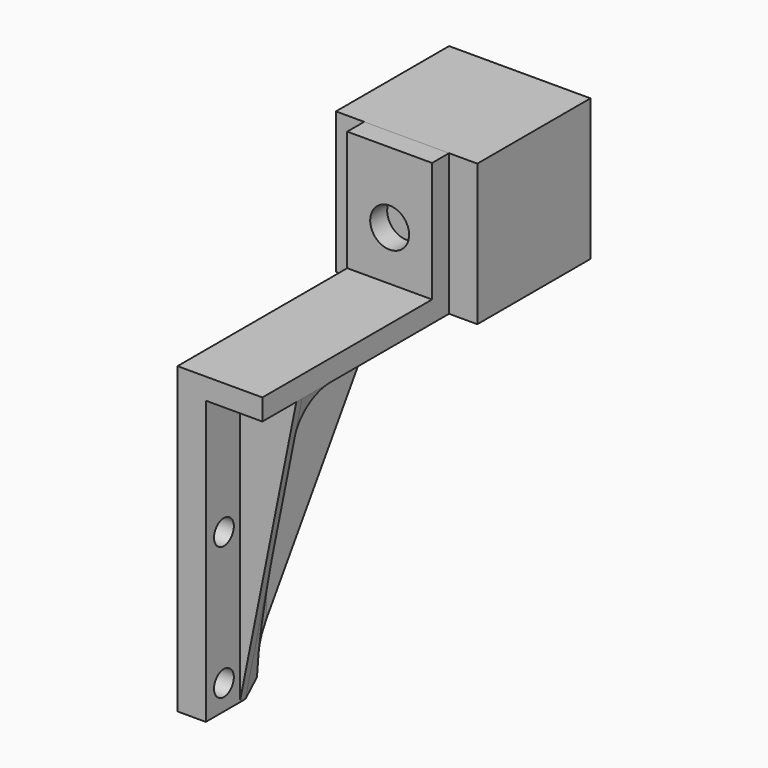
from build123d import *

# Parameters (mm, degrees)
F0_W          = 20
F0_H          = 20
F1_DEPTH      = 20
F2_W          = 12
F2_H          = 20
F2_R          = 2.75
F3_DEPTH      = 3
F4_W          = 12
F4_H          = 3
F5_DEPTH      = 30
F6_W          = 4
F6_H          = 7
F7_DEPTH      = 40
F8_R          = 1.75
F9_DEPTH      = 25
F11_DEPTH     = 1
F12_W         = 3
F12_H         = 6
F13_DEPTH     = 2
F15_DEPTH     = 3
F16_S3_W      = 5
F16_S3_H      = 5
F16_T4_DEPTH  = 5
F16_T10_DEPTH = 21
F16_T15_DEPTH = 4
F16_T20_DEPTH = 35


# Not quite as in the source:
# - a fillet or chamfer that OpenCascade refuses, or shapes differently, is made with other operations: its cross-section is extruded or revolved along the edge and cut away or added


with BuildPart() as f1:
    # F0 (on Right) → F1 (new body)
    with BuildSketch(Plane.YZ):
        Rectangle(F0_W, F0_H)
    extrude(amount=F1_DEPTH)


with BuildPart() as f3:
    # F2 (on face) → F3 (new body)
    with BuildSketch(Plane.XZ.offset(10)):
        with Locations((10, 0)):
            Rectangle(F2_W, F2_H)
        with Locations((10, 0)):
            Circle(F2_R, mode=Mode.SUBTRACT)
    extrude(amount=F3_DEPTH)

    # F4 (on face) → F5 (join)
    with BuildSketch(Plane.XZ.offset(13)):
        with Locations((10, -8.5)):
            Rectangle(F4_W, F4_H)
    extrude(amount=F5_DEPTH)

    # F6 (on face) → F7 (join)
    with BuildSketch(Plane(origin=(0, 0, -10), x_dir=(1, 0, 0), z_dir=(0, 0, -1))):
        with Locations((6, 39.5)):
            Rectangle(F6_W, F6_H)
    extrude(amount=F7_DEPTH)

    # F8 (on face) → F9 (cut)
    with BuildSketch(Plane.YZ.offset(8)):
        with Locations((-39.8, -46.45)):
            Circle(F8_R)
        with Locations((-39.8, -27.65)):
            Circle(F8_R)
    extrude(amount=-F9_DEPTH, mode=Mode.SUBTRACT)

    # F10 (on face) → F11 (join)
    with BuildSketch(Plane(origin=(0, -36, 0), x_dir=(-1, 0, 0), z_dir=(0, 1, 0))):
        Polygon((-16, -10), (-8, -50), (-8, -10), align=None)
    extrude(amount=-F11_DEPTH)

    # F12 (on face) → F13 (cut)
    with BuildSketch(Plane(origin=(4, 0, 0), x_dir=(0, -1, 0), z_dir=(-1, 0, 0))):
        with Locations((37.5, -20)):
            Rectangle(F12_W, F12_H)
    extrude(amount=-F13_DEPTH, mode=Mode.SUBTRACT)

    # F14 (on face) → F15 (join)
    with BuildSketch(Plane(origin=(4, 0, 0), x_dir=(0, -1, 0), z_dir=(-1, 0, 0))):
        Polygon((36, -17), (36, -10), (10, -10), (36, -50), (36, -23), align=None)
    extrude(amount=-F15_DEPTH)

    # F16: fillet of radius 5 on 3 edges, made by hand


with BuildPart() as f16_tool2:
    # F16_s3 → F16_t4 (new body)
    with BuildSketch(Plane.XY.offset(-15)):
        with Locations((9.5, -33.5)):
            Rectangle(F16_S3_W, F16_S3_H)
    extrude(amount=F16_T4_DEPTH)

    # F16_s5 → F16_t6 (revolve, cut)
    with BuildSketch(Plane(origin=(12, -31, -15), x_dir=(0.7071067812, 0.7071067812, 0), z_dir=(0.7071067812, -0.7071067812, 0))):
        with BuildLine():
            ThreePointArc((0, -5), (5, 0), (0, 5))
            Line((0, 5), (0, -5))
        make_face()
    revolve(axis=Axis((12, -31, -15), (0, 0, 1)), mode=Mode.SUBTRACT)


with BuildPart() as f3_1:
    add(f3.part)

    # F16_t1: union F16_tool2
    add(f16_tool2.part)


with BuildPart() as f16_tool8:
    # F16_s9 → F16_t10 (new body)
    with BuildSketch(Plane.XZ.offset(31)):
        with BuildLine():
            ThreePointArc((12, -10), (8.4644660941, -11.4644660941), (7, -15))
            Line((7, -15), (7, -10))
            Line((7, -10), (12, -10))
        make_face()
    extrude(amount=-F16_T10_DEPTH)

    split(bisect_by=Plane(origin=(0, -2.460456942, 1.5992970123), x_dir=(1, 0, 0), z_dir=(0, -0.8384436163, 0.5449883506)), keep=Keep.TOP)


with BuildPart() as f3_2:
    add(f3_1.part)

    # F16_t7: union F16_tool8
    add(f16_tool8.part)


with BuildPart() as f16_tool13:
    # F16_s14 → F16_t15 (new body)
    with BuildSketch(Plane.YZ.offset(16)):
        with BuildLine():
            ThreePointArc((-31, -10), (-34.5355339059, -11.4644660941), (-36, -15))
            Line((-36, -15), (-36, -10))
            Line((-36, -10), (-31, -10))
        make_face()
    extrude(amount=-F16_T15_DEPTH)

    split(bisect_by=Plane(origin=(17.3076923077, 0, -3.4615384615), x_dir=(0, 1, 0), z_dir=(-0.9805806757, 0, 0.1961161351)), keep=Keep.TOP)


with BuildPart() as f3_3:
    add(f3_2.part)

    # F16_t12: union F16_tool13
    add(f16_tool13.part)


with BuildPart() as f16_tool18:
    # F16_s19 → F16_t20 (new body)
    with BuildSketch(Plane.XY.offset(-50)):
        with BuildLine():
            ThreePointArc((7, -31), (8.4644660941, -34.5355339059), (12, -36))
            Line((12, -36), (7, -36))
            Line((7, -36), (7, -31))
        make_face()
    extrude(amount=F16_T20_DEPTH)

    split(bisect_by=Plane(origin=(0, -2.460456942, 1.5992970123), x_dir=(1, 0, 0), z_dir=(0, -0.8384436163, 0.5449883506)), keep=Keep.TOP)

    split(bisect_by=Plane(origin=(17.3076923077, 0, -3.4615384615), x_dir=(0, 1, 0), z_dir=(-0.9805806757, 0, 0.1961161351)), keep=Keep.TOP)


with BuildPart() as f3_4:
    add(f3_3.part)

    # F16_t17: union F16_tool18
    add(f16_tool18.part)


solid = Compound([f1.part, f3_4.part])
